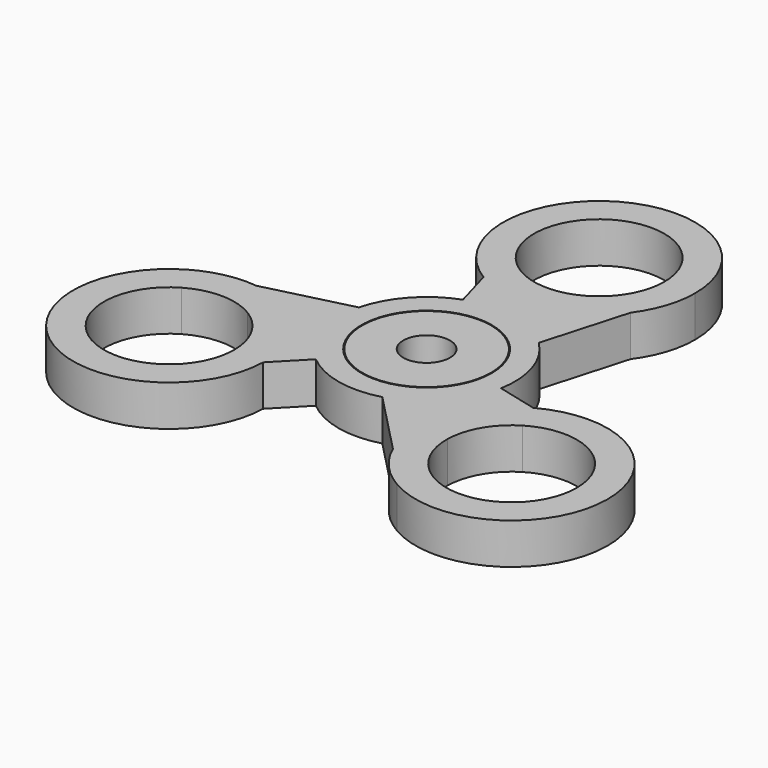
from build123d import *

# Parameters (mm, degrees)
F0_R            = 11
F0_R_2          = 4
F1_DEPTH        = 7
F2_R            = 15.0849931144
F2_R_2          = 11.15
F3_DEPTH        = 7
F5_DEPTH        = 7
F5_COPIES_COUNT = 3


# Not quite as in the source:
# - a pattern or mirror of a feature is missing from the dataset's text; its kind, count and spacing are read off the source's solid


with BuildPart() as f1:
    # F0 (on Top) → F1 (new body)
    with BuildSketch(Plane.XY):
        Circle(F0_R)
        Circle(F0_R_2, mode=Mode.SUBTRACT)
    extrude(amount=F1_DEPTH)


with BuildPart() as f3:
    # F2 (on Top) → F3 (new body)
    with BuildSketch(Plane.XY):
        Circle(F2_R)
        Circle(F2_R_2, mode=Mode.SUBTRACT)
    extrude(amount=F3_DEPTH)

    # F4 (on Top) → F5 (join)
    with BuildSketch(Plane.XY):
        with BuildLine():
            Line((-7.0745577316, 21.0109236638), (-4.8416383778, 13.1369449955))
            Line((-4.8416383778, 13.1369449955), (6.196208957, 12.7750489976))
            Line((6.196208957, 12.7750489976), (9.9961235482, 8.7941850849))
            Line((9.9961235482, 8.7941850849), (14.7007794568, 25.2604825284))
            ThreePointArc((14.7007794568, 25.2604825284), (4.6386657732, 18.9054436461), (-7.0745577316, 21.0109236638))
        make_face()
        with BuildLine():
            ThreePointArc((17.9220181184, 35.0316912253), (-6.5463257275, 49.361823179), (-7.0745577316, 21.0109236638))
            Line((-7.0745577316, 21.0109236638), (-8.2796565302, 25.2604825284))
            Line((-8.2796565302, 25.2604825284), (-3.8792922685, 25.2604825284))
            ThreePointArc((-3.8792922685, 25.2604825284), (-4.184606348, 44.6287591763), (12.6415531586, 35.0316912253))
            ThreePointArc((12.6415531586, 35.0316912253), (11.0886211095, 29.3555317188), (6.8623985856, 25.2604825284))
            Line((6.8623985856, 25.2604825284), (14.7007794568, 25.2604825284))
            ThreePointArc((14.7007794568, 25.2604825284), (17.0959421027, 29.8874493494), (17.9220181184, 35.0316912253))
        make_face()
        with BuildLine():
            Line((-8.2796565302, 25.2604825284), (-7.0745577316, 21.0109236638))
            ThreePointArc((-7.0745577316, 21.0109236638), (4.6386657732, 18.9054436461), (14.7007794568, 25.2604825284))
            Line((14.7007794568, 25.2604825284), (6.8623985856, 25.2604825284))
            ThreePointArc((6.8623985856, 25.2604825284), (1.4915531586, 23.8816912253), (-3.8792922685, 25.2604825284))
            Line((-3.8792922685, 25.2604825284), (-8.2796565302, 25.2604825284))
        make_face()
    f5 = extrude(amount=F5_DEPTH)

    # F5_copies: F5 ×3 about axis
    f5_copies_axis = Axis((0, 0, 0), (0, 0, 1))
    for i in range(1, F5_COPIES_COUNT):
        add(f5.rotate(f5_copies_axis, i * 360 / F5_COPIES_COUNT))


solid = Compound([f1.part, f3.part])
